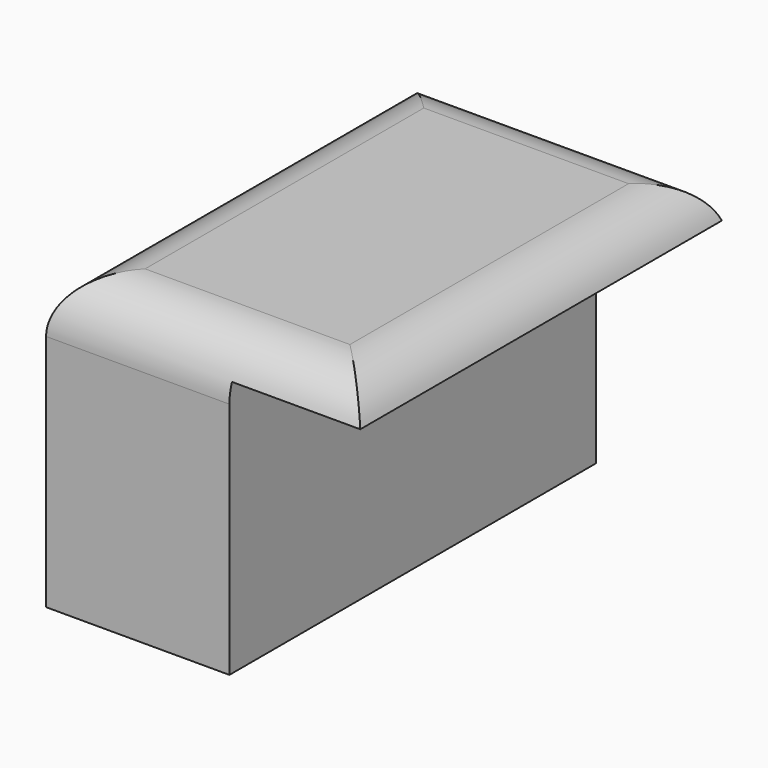
from build123d import *

# Parameters (mm, degrees)
F0_W        = 4
F0_H        = 3.5
F1_DEPTH    = 16
F2_START    = 14
F0_W_2      = 7
F0_H_2      = 25
F2_DEPTH    = 2
F3_START    = 4.485
F3_DEPTH    = 4
F4_T1_DEPTH = 40
F4_T3_DEPTH = 32
F4_T5_DEPTH = 39.1421356237


# Not quite as in the source:
# - a fillet or chamfer that OpenCascade refuses, or shapes differently, is made with other operations: its cross-section is extruded or revolved along the edge and cut away or added


with BuildPart() as f1:
    # F0 (on Top) → F1 (new body)
    with BuildSketch(Plane.XY):
        Polygon((-6.5023180035, -17.3460646598), (3.4976819965, -17.3460646598), (3.4976819965, 7.6539353402), (-0.0023180035, 7.6539353402), (-0.0023180035, 4.1539353402), (-4.0023180035, 4.1539353402), (-4.0023180035, 7.6539353402), (-6.5023180035, 7.6539353402), align=None)
        with Locations((-2.0023180035, 5.9039353402)):
            Rectangle(F0_W, F0_H)
    extrude(amount=F1_DEPTH)

    # F0 (on Top) → F2 (join)
    with BuildSketch(Plane.XY.offset(F2_START)):
        with Locations((6.9976819965, -4.8460646598)):
            Rectangle(F0_W_2, F0_H_2)
    extrude(amount=F2_DEPTH)

    # F0 (on Top) → F3 (cut)
    with BuildSketch(Plane.XY.offset(F3_START)):
        with Locations((-2.0023180035, 5.9039353402)):
            Rectangle(F0_W, F0_H)
    extrude(amount=F3_DEPTH, mode=Mode.SUBTRACT)

    # F4: fillet of radius 3 on 4 edges, made by hand

    # F4_s2 → F4_t1 (cut)
    with BuildSketch(Plane.XZ.offset(-15.1539353402)):
        with BuildLine():
            ThreePointArc((-6.5023180035, 13), (-5.6236383471, 15.1213203436), (-3.5023180035, 16))
            Line((-3.5023180035, 16), (-6.5023180035, 16))
            Line((-6.5023180035, 16), (-6.5023180035, 13))
        make_face()
    extrude(amount=F4_T1_DEPTH, mode=Mode.SUBTRACT)

    # F4_s4 → F4_t3 (cut)
    with BuildSketch(Plane.YZ.offset(-14.0023180035)):
        with BuildLine():
            ThreePointArc((-17.3460646598, 13), (-16.4673850034, 15.1213203436), (-14.3460646598, 16))
            Line((-14.3460646598, 16), (-17.3460646598, 16))
            Line((-17.3460646598, 16), (-17.3460646598, 13))
        make_face()
        with BuildLine():
            ThreePointArc((7.6539353402, 13), (6.7752556838, 15.1213203436), (4.6539353402, 16))
            Line((4.6539353402, 16), (7.6539353402, 16))
            Line((7.6539353402, 16), (7.6539353402, 13))
        make_face()
    extrude(amount=F4_T3_DEPTH, mode=Mode.SUBTRACT)

    # F4_s6 → F4_t5 (cut)
    with BuildSketch(Plane.XZ.offset(-14.7250031521)):
        with BuildLine():
            ThreePointArc((7.6692548718, 16), (9.4013056793, 15.4494897428), (10.4976819965, 14))
            Line((10.4976819965, 14), (10.4976819965, 16))
            Line((10.4976819965, 16), (7.6692548718, 16))
        make_face()
    extrude(amount=F4_T5_DEPTH, mode=Mode.SUBTRACT)


solid = f1.part
